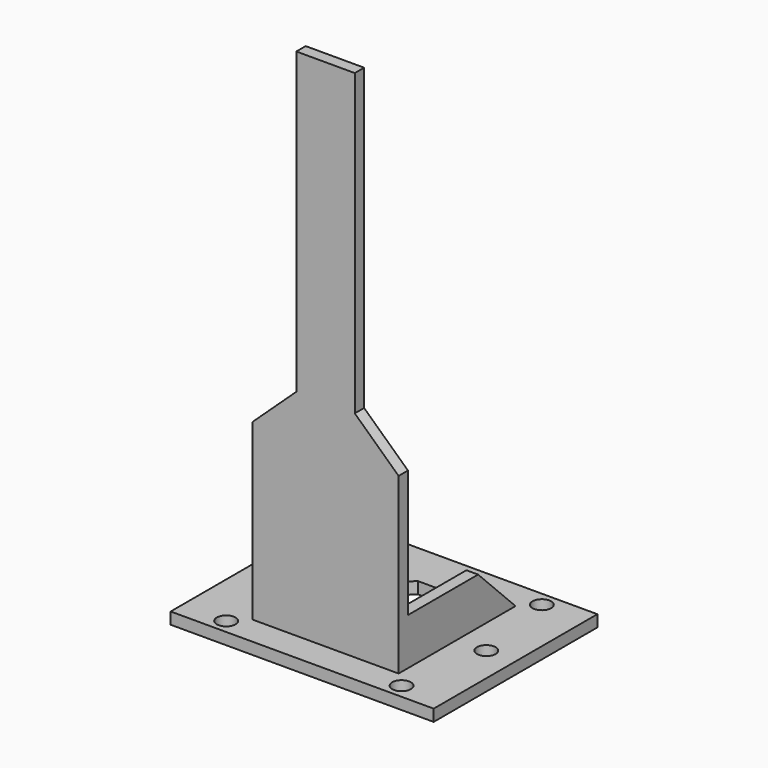
from build123d import *

# Parameters (mm, degrees)
F1_W     = 21
F1_H     = 21
F1_R     = 1.1
F1_H_2   = 2
F1_W_2   = 10
F1_H_3   = 15
F1_R_2   = 1.6
F2_DEPTH = 2
F3_DEPTH = 90
F4_DEPTH = 10
F5_SIZE  = 7.99999
F7_DEPTH = 25


# Not quite as in the source:
# - a fillet or chamfer is up to 0.001 mm smaller than in the source, because OpenCascade refuses the exact size


with BuildPart() as f2:
    # F1 (on Top) → F2 (new body)
    with BuildSketch(Plane.XY):
        Rectangle(F1_W, F1_H)
        with Locations((-8, -8)):
            Circle(F1_R, mode=Mode.SUBTRACT)
        with Locations((8, -8)):
            Circle(F1_R, mode=Mode.SUBTRACT)
        with Locations((-8, 8)):
            Circle(F1_R, mode=Mode.SUBTRACT)
        Polygon((-10, 2.2218254069), (-2.2218254069, 10), (2.2218254069, 10), (10, 2.2218254069), (10, -2.2218254069), (2.2218254069, -10), (-2.2218254069, -10), (-10, -2.2218254069), align=None, mode=Mode.SUBTRACT)
        with Locations((8, 8)):
            Circle(F1_R, mode=Mode.SUBTRACT)
        Polygon((-10.5, 12.5), (-12.5, 12.5), (-12.5, 7.8503944539), (-12.5, -7.1496055461), (-12.5, -10.5), (-10.5, -10.5), (-10.5, 10.5), align=None)
        with Locations((0, 11.5)):
            Rectangle(F1_W, F1_H_2)
        Polygon((12.5, 12.5), (10.5, 12.5), (10.5, 10.5), (10.5, -10.5), (12.5, -10.5), (12.5, -7.1496055461), (12.5, 7.8503944539), align=None)
        with Locations((-17.5, 0.3503944539)):
            Rectangle(F1_W_2, F1_H_3)
        with Locations((-17.5, 0)):
            Circle(F1_R_2, mode=Mode.SUBTRACT)
        with Locations((17.5, 0.3503944539)):
            Rectangle(F1_W_2, F1_H_3)
        with Locations((17.5, 0)):
            Circle(F1_R_2, mode=Mode.SUBTRACT)
        Polygon((-12.5, 7.8503944539), (-12.5, 12.5), (-10.5, 12.5), (10.5, 12.5), (12.5, 12.5), (12.5, 7.8503944539), (22.5, 7.8503944539), (22.5, 17.5), (-22.5, 17.5), (-22.5, 7.8503944539), align=None)
        with Locations((-15, 15)):
            Circle(F1_R_2, mode=Mode.SUBTRACT)
        with Locations((15, 15)):
            Circle(F1_R_2, mode=Mode.SUBTRACT)
        Polygon((-12.5, -10.5), (-12.5, -7.1496055461), (-22.5, -7.1496055461), (-22.5, -17.5), (22.5, -17.5), (22.5, -7.1496055461), (12.5, -7.1496055461), (12.5, -10.5), (12.5, -12.5), (-12.5, -12.5), align=None)
        with Locations((-15, -15)):
            Circle(F1_R_2, mode=Mode.SUBTRACT)
        with Locations((15, -15)):
            Circle(F1_R_2, mode=Mode.SUBTRACT)
        Polygon((10.5, -10.5), (-10.5, -10.5), (-12.5, -10.5), (-12.5, -12.5), (12.5, -12.5), (12.5, -10.5), align=None)
    extrude(amount=F2_DEPTH)

    # F1 (on Top) → F3 (join)
    with BuildSketch(Plane.XY):
        Polygon((10.5, -10.5), (-10.5, -10.5), (-12.5, -10.5), (-12.5, -12.5), (12.5, -12.5), (12.5, -10.5), align=None)
    extrude(amount=F3_DEPTH)

    # F1 (on Top) → F4 (join)
    with BuildSketch(Plane.XY):
        Polygon((12.5, 12.5), (10.5, 12.5), (10.5, 10.5), (10.5, -10.5), (12.5, -10.5), (12.5, -7.1496055461), (12.5, 7.8503944539), align=None)
        Polygon((-10.5, 12.5), (-12.5, 12.5), (-12.5, 7.8503944539), (-12.5, -7.1496055461), (-12.5, -10.5), (-10.5, -10.5), (-10.5, 10.5), align=None)
        Polygon((10.5, -10.5), (-10.5, -10.5), (-12.5, -10.5), (-12.5, -12.5), (12.5, -12.5), (12.5, -10.5), align=None)
    extrude(amount=F4_DEPTH)

    # F5 (size 8 in the source; OpenCascade refuses exactly that, so slightly less here)
    f5_edges = [f2.edges().sort_by_distance(p)[0] for p in [
        (11.5, 12.5, 10),
        (-11.5, 12.5, 10),
    ]]
    chamfer(f5_edges, length=F5_SIZE)

    # F6 (on face) → F7 (cut)
    with BuildSketch(Plane(origin=(0, -10.5, 0), x_dir=(-1, 0, 0), z_dir=(0, 1, 0))):
        Polygon((-12.5, 90), (-12.5, 31.766526401), (-5, 38.7480794755), (-5, 90), align=None)
        Polygon((5, 38.7480794755), (12.5, 31.766526401), (12.5, 90), (5, 90), align=None)
    extrude(amount=-F7_DEPTH, mode=Mode.SUBTRACT)


solid = f2.part
